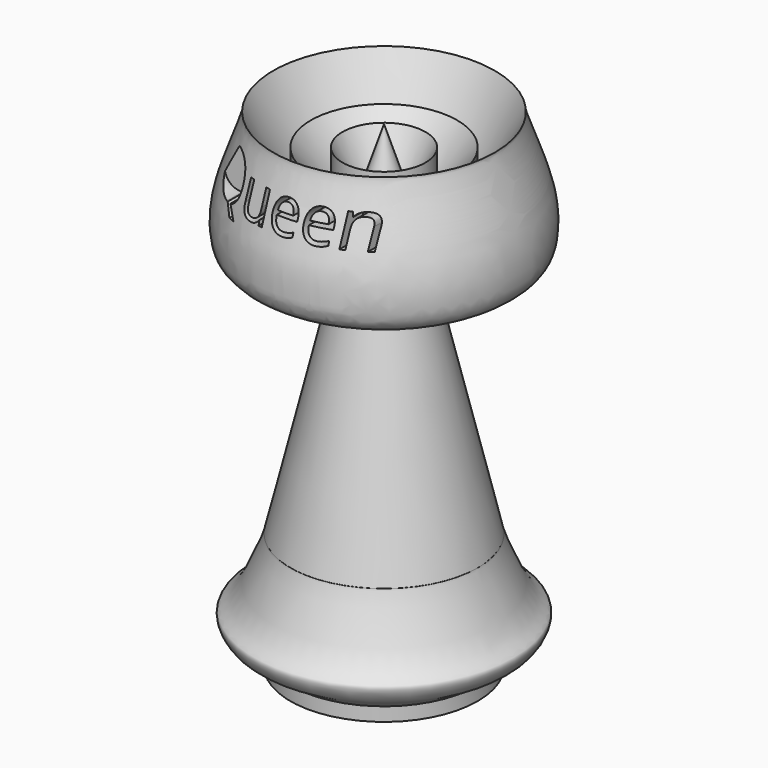
from build123d import *

# Parameters (mm, degrees)
F3_TEXT_SIZE = 11.5651039052
F4_DEPTH     = 19.8


# Not quite as in the source:
# - Text() gives the source's letters only with a copy of the font that has no kerning and outlines rounded to 1/6400 em; it was checked with that copy


with BuildPart() as f1:
    # F0 (on Front) → F1 (revolve)
    with BuildSketch(Plane.XZ):
        with BuildLine():
            Line((4.2728638967, 32.9334698617), (0, 45.9979847074))
            Line((0, 45.9979847074), (0, -55.2520155907))
            Line((0, -55.2520155907), (19.8689512908, -55.2520155907))
            Line((19.8689512908, -55.2520155907), (19.8689512908, -52.3487925529))
            add(Edge.make_bspline(
                [(19.8689512908, -52.3487925529), (20.5261000959, -51.847988848), (21.847389856, -50.8410528206), (24.0623458375, -49.5911124849), (26.7749399951, -48.2279352879), (28.4315273711, -44.2972830016), (24.4882932202, -43.7072514397), (19.7375561435, -30.6922348602), (19.8564547872, -30.4215912092), (19.8689512908, -30.3931459785)],
                knots=[0, 0, 0, 0, 0.1250207587, 0.2513717548, 0.3919804389, 0.5321117418, 0.6774629004, 0.966100656, 1, 1, 1, 1], degree=3))
            Line((19.8689512908, -30.3931459785), (7.8931450844, 19.8689512908))
            Line((7.8931450844, 19.8689512908), (23.4979856759, 19.8689512908))
            add(Edge.make_bspline(
                [(23.4979856759, 19.8689512908), (25.0385762625, 20.6132894157), (27.9367181302, 22.0135300132), (28.9939209043, 25.9435515588), (28.8407917676, 31.6005561354), (26.9784695102, 37.7521949184), (25.0985675038, 42.7943392542), (23.3984225948, 47.687834383), (23.5009922551, 48.1302412829), (23.5010275228, 48.2559515428), (23.5000248721, 48.2960566225)],
                knots=[0, 0, 0, 0, 0.1485368589, 0.2794258861, 0.4414205861, 0.6139247279, 0.7807507908, 0.9297767818, 0.9709127656, 0.9902321409, 0.9902321409, 0.9902321409, 0.9902321409], degree=3))
            Line((23.5000248721, 48.2960566225), (15.5141139403, 32.9334698617))
            Line((15.5141139403, 32.9334698617), (15.5141139403, 41.6431464255))
            Line((15.5141139403, 41.6431464255), (8.8004022837, 32.9334698617))
            Line((8.8004022837, 32.9334698617), (8.8004022837, 41.6431464255))
            Line((8.8004022837, 41.6431464255), (4.2728638967, 32.9334698617))
        make_face()
    revolve(axis=Axis((0, 0, -4.6270154417), (0, 0, -1)))

    # F3 (on offset) → F4 (cut)
    with BuildSketch(Plane.XZ.offset(38.8)):
        with Locations((-19.3790479351, 36.3067562646)):
            Text('Queen', F3_TEXT_SIZE, font='Open Sans', text_align=(TextAlign.LEFT, TextAlign.BOTTOM))
        with BuildLine():
            add(Edge.make_bspline(
                [(-16.9422444014, 42.967533295), (-17.6569316818, 42.1001505021), (-17.6569316818, 40.4467020532)],
                knots=[0, 0, 0, 1, 1, 1], degree=2))
            add(Edge.make_bspline(
                [(-17.6569316818, 40.4467020532), (-17.6569316818, 38.7697619869), (-16.9422444014, 37.902379194)],
                knots=[0, 0, 0, 1, 1, 1], degree=2))
            add(Edge.make_bspline(
                [(-16.9422444014, 37.902379194), (-16.227557121, 37.0349964011), (-14.8668503646, 37.0349964011)],
                knots=[0, 0, 0, 1, 1, 1], degree=2))
            add(Edge.make_bspline(
                [(-14.8668503646, 37.0349964011), (-13.4953013234, 37.0349964011), (-12.7950704229, 37.898765099)],
                knots=[0, 0, 0, 1, 1, 1], degree=2))
            add(Edge.make_bspline(
                [(-12.7950704229, 37.898765099), (-12.0948395223, 38.762533797), (-12.0948395223, 40.4467020532)],
                knots=[0, 0, 0, 1, 1, 1], degree=2))
            add(Edge.make_bspline(
                [(-12.0948395223, 40.4467020532), (-12.0948395223, 42.1127998345), (-12.7923598516, 42.9738579612)],
                knots=[0, 0, 0, 1, 1, 1], degree=2))
            add(Edge.make_bspline(
                [(-12.7923598516, 42.9738579612), (-13.4898801809, 43.8349160879), (-14.8560080797, 43.8349160879)],
                knots=[0, 0, 0, 1, 1, 1], degree=2))
            add(Edge.make_bspline(
                [(-14.8560080797, 43.8349160879), (-16.227557121, 43.8349160879), (-16.9422444014, 42.967533295)],
                knots=[0, 0, 0, 1, 1, 1], degree=2))
        make_face()
    extrude(amount=-F4_DEPTH, mode=Mode.SUBTRACT)


solid = f1.part
